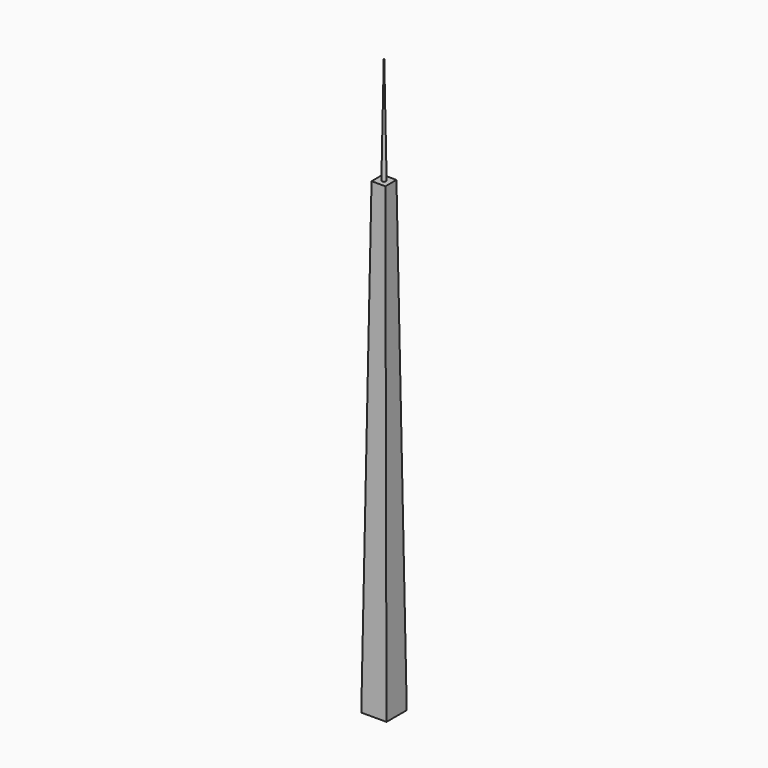
from build123d import *

# Parameters (mm, degrees)
F0_W     = 54.1937425733
F0_H     = 54.301276803
F1_DEPTH = 1003.3
F1_TAPER = 0.7
F2_R     = 4.4355326491
F3_DEPTH = 630.428
F3_TAPER = 1


# Not quite as in the source:
# - a feature names something its author has since deleted; it is built from what else it names


with BuildPart() as f1:
    # F0 (on Top) → F1 (new body)
    with BuildSketch(Plane.XY):
        Rectangle(F0_W, F0_H)
    extrude(amount=F1_DEPTH, taper=F1_TAPER)

    # F2 (on face) → F3 (join)
    with BuildSketch(Plane.XY.offset(1003.3)):
        Circle(F2_R)
    extrude(amount=F3_DEPTH, taper=F3_TAPER)


solid = f1.part
